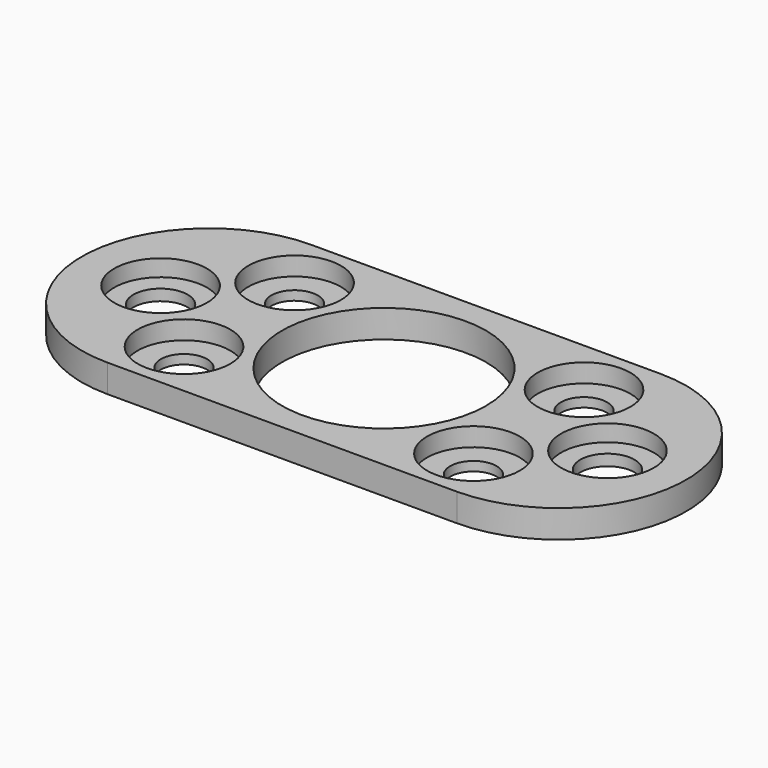
from build123d import *

# Parameters (mm, degrees)
F0_R           = 11
F1_DEPTH       = 3
F2_D           = 5.85
F2_CBORE_D     = 10
F2_CBORE_DEPTH = 1.8
F3_D           = 5
F3_CBORE_D     = 10
F3_CBORE_DEPTH = 2


# Not quite as in the source:
# - a feature names something its author has since deleted; it is built from what else it names


with BuildPart() as f1:
    # F0 (on Top) → F1 (new body)
    with BuildSketch(Plane.XY):
        with BuildLine():
            Line((18.85, 13.75), (-18.85, 13.75))
            ThreePointArc((-18.85, 13.75), (-32.6, 0), (-18.85, -13.75))
            Line((-18.85, -13.75), (18.85, -13.75))
            ThreePointArc((18.85, -13.75), (32.6, 0), (18.85, 13.75))
        make_face()
        Circle(F0_R, mode=Mode.SUBTRACT)
    extrude(amount=-F1_DEPTH)

    # F2 (through all)
    with Locations(Plane.XY):
        with Locations((24.1, 0), (-24.1, 0)):
            CounterBoreHole(F2_D / 2, F2_CBORE_D / 2, F2_CBORE_DEPTH)

    # F3 (through all)
    with Locations(Plane.XY):
        with Locations((-15.6095083693, 7.4526413832), (-15.6095083693, -7.4526413832), (15.6095083693, -7.4526413832), (15.6095083693, 7.4526413832)):
            CounterBoreHole(F3_D / 2, F3_CBORE_D / 2, F3_CBORE_DEPTH)


solid = f1.part
